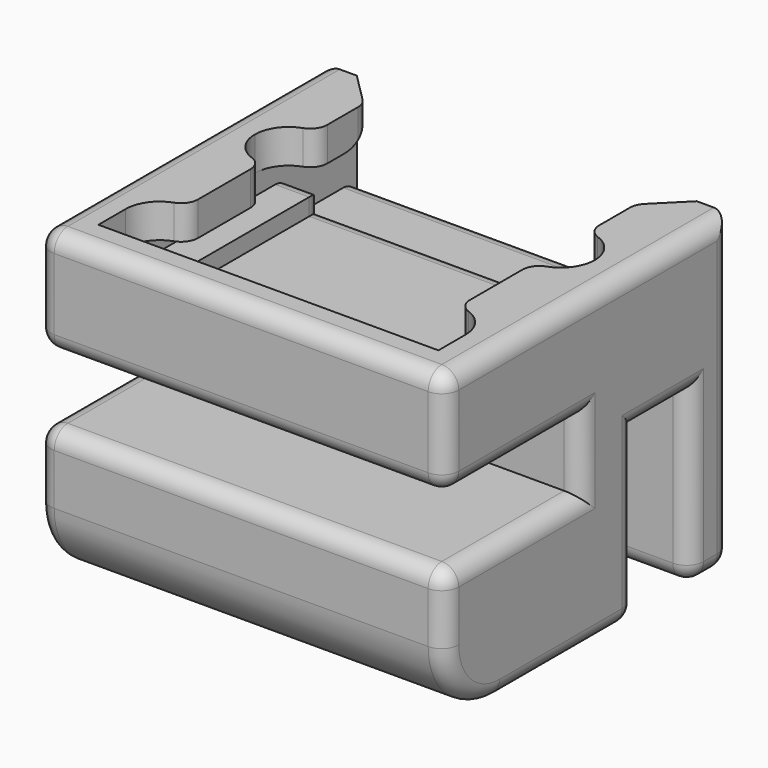
from build123d import *

# Parameters (mm, degrees)
F0_W           = 30.48
F0_H           = 26.67
F1_DEPTH       = 19.05
F3_DEPTH       = 1.524
F5_DEPTH       = 2.54
F6_W           = 20.32
F6_H           = 24.13
F7_DEPTH       = 1.27
F8_W           = 25.4
F8_H           = 6.35
F9_DEPTH       = 2.794
F10_W          = 12.7
F10_H          = 5.08
F10_W_2        = 5.08
F10_H_2        = 12.7
F11_DEPTH      = 30.481
F12_R          = 5.08
F13_T1_DEPTH   = 27.94
F13_T3_DEPTH   = 3.81
F13_T5_DEPTH   = 11.43
F13_T7_DEPTH   = 11.43
F13_T9_DEPTH   = 5.08
F13_T11_DEPTH  = 11.43
F13_T13_DEPTH  = 5.08
F13_T15_DEPTH  = 5.334
F13_T17_DEPTH  = 25.4
F13_T19_DEPTH  = 1.27
F13_T21_DEPTH  = 21.844
F13_T23_DEPTH  = 25.4
F13_T25_DEPTH  = 20.32
F13_T27_DEPTH  = 2.54
F13_T29_DEPTH  = 1.27
F13_T31_DEPTH  = 2.54
F13_T33_DEPTH  = 2.54
F13_S37_W      = 1.2954
F13_S37_H      = 1.2954
F13_T38_DEPTH  = 1.2954
F13_S43_W      = 1.2954
F13_S43_H      = 1.2954
F13_T44_DEPTH  = 1.2954
F13_S49_W      = 1.2954
F13_S49_H      = 1.2954
F13_T50_DEPTH  = 1.2954
F13_S55_W      = 1.2954
F13_S55_H      = 1.2954
F13_T56_DEPTH  = 1.2954
F13_S61_W      = 1.2954
F13_S61_H      = 1.2954
F13_T62_DEPTH  = 1.2954
F13_S67_W      = 1.2954
F13_S67_H      = 1.2954
F13_T68_DEPTH  = 1.2954
F13_S73_W      = 1.2954
F13_S73_H      = 1.2954
F13_T74_DEPTH  = 1.2954
F13_S79_W      = 1.2954
F13_S79_H      = 1.2954
F13_T80_DEPTH  = 1.2954
F13_S85_W      = 1.2954
F13_S85_H      = 1.2954
F13_T86_DEPTH  = 1.2954
F13_S91_W      = 1.2954
F13_S91_H      = 1.2954
F13_T92_DEPTH  = 1.2954
F13_S97_W      = 1.2954
F13_S97_H      = 1.2954
F13_T98_DEPTH  = 1.2954
F13_S103_W     = 1.2954
F13_S103_H     = 1.2954
F13_T104_DEPTH = 1.2954
F13_T108_ANGLE = 90
F13_T110_ANGLE = 90
F13_T114_DEPTH = 9.9421024484
F13_T121_DEPTH = 9.9421024484
F13_T129_DEPTH = 14.605
F13_T133_DEPTH = 8.255
F13_T140_DEPTH = 8.255
F13_T144_DEPTH = 14.605
F13_T151_DEPTH = 14.605
F13_T155_DEPTH = 8.255
F13_T162_DEPTH = 8.255
F13_T166_DEPTH = 14.605
F13_T173_DEPTH = 28.575
F13_T177_DEPTH = 25.019
F13_T184_DEPTH = 14.605
F13_T188_DEPTH = 8.255
F13_T195_DEPTH = 8.255
F13_T199_DEPTH = 14.605
F13_T206_DEPTH = 14.605
F13_T210_DEPTH = 8.255
F13_T217_DEPTH = 8.255
F13_T221_DEPTH = 14.605
F13_T228_DEPTH = 28.575
F13_T232_DEPTH = 25.019
F13_T239_DEPTH = 4.445
F13_T243_DEPTH = 23.495
F13_T250_DEPTH = 23.495
F13_T254_DEPTH = 4.445
F13_T261_DEPTH = 5.715
F13_T265_DEPTH = 4.445
F13_T272_DEPTH = 5.715
F13_T276_DEPTH = 4.445
F13_T283_DEPTH = 3.8551280605
F13_T287_DEPTH = 9.9421024484
F13_T294_DEPTH = 3.8551280605
F13_T298_DEPTH = 9.9421024484


# Not quite as in the source:
# - a fillet or chamfer that OpenCascade refuses, or shapes differently, is made with other operations: its cross-section is extruded or revolved along the edge and cut away or added


with BuildPart() as f1:
    # F0 (on Top) → F1 (new body)
    with BuildSketch(Plane.XY):
        Rectangle(F0_W, F0_H)
    extrude(amount=F1_DEPTH)

    # F2 (on face) → F3 (join)
    with BuildSketch(Plane.XY.offset(19.05)):
        Polygon((-12.7, 13.335), (-15.24, 13.335), (-15.24, -13.335), (15.24, -13.335), (15.24, 13.335), (12.7, 13.335), (12.7, -10.795), (-12.7, -10.795), align=None)
    extrude(amount=F3_DEPTH)

    # F4 (on face) → F5 (join)
    with BuildSketch(Plane.XY.offset(20.574)):
        with BuildLine():
            ThreePointArc((-10.16, 1.27), (-11.9560512242, 2.0139487758), (-12.7, 3.81))
            Line((-12.7, 3.81), (-12.7, -8.255))
            ThreePointArc((-12.7, -8.255), (-11.9560512242, -6.4589487758), (-10.16, -5.715))
            Line((-10.16, -5.715), (-10.16, 1.27))
        make_face()
        with BuildLine():
            Line((-10.16, 10.795), (-12.7, 13.335))
            Line((-12.7, 13.335), (-12.7, 3.81))
            ThreePointArc((-12.7, 3.81), (-11.9560512242, 5.6060512242), (-10.16, 6.35))
            Line((-10.16, 6.35), (-10.16, 10.795))
        make_face()
        Polygon((15.24, -13.335), (15.24, 13.335), (12.7, 13.335), (12.7, 3.81), (12.7, -8.255), (12.7, -10.795), (0, -10.795), (-12.7, -10.795), (-12.7, -8.255), (-12.7, 3.81), (-12.7, 13.335), (-15.24, 13.335), (-15.24, -13.335), align=None)
        with BuildLine():
            Line((12.7, -8.255), (12.7, 3.81))
            ThreePointArc((12.7, 3.81), (11.9560512242, 2.0139487758), (10.16, 1.27))
            Line((10.16, 1.27), (10.16, -5.715))
            ThreePointArc((10.16, -5.715), (11.9560512242, -6.4589487758), (12.7, -8.255))
        make_face()
        with BuildLine():
            Line((12.7, 3.81), (12.7, 13.335))
            Line((12.7, 13.335), (10.16, 10.795))
            Line((10.16, 10.795), (10.16, 6.35))
            ThreePointArc((10.16, 6.35), (11.9560512242, 5.6060512242), (12.7, 3.81))
        make_face()
    extrude(amount=F5_DEPTH)

    # F6 (on face) → F7 (cut)
    with BuildSketch(Plane.XY.offset(19.05)):
        with Locations((0, 1.27)):
            Rectangle(F6_W, F6_H)
    extrude(amount=-F7_DEPTH, mode=Mode.SUBTRACT)

    # F8 (on face) → F9 (cut)
    with BuildSketch(Plane.XY.offset(19.05)):
        with Locations((0, 10.16)):
            Rectangle(F8_W, F8_H)
    extrude(amount=-F9_DEPTH, mode=Mode.SUBTRACT)

    # F10 (on face) → F11 (cut, through all)
    with BuildSketch(Plane.YZ.offset(15.24)):
        with Locations((-6.985, 12.7)):
            Rectangle(F10_W, F10_H)
        with Locations((6.985, 6.35)):
            Rectangle(F10_W_2, F10_H_2)
    extrude(amount=-F11_DEPTH, mode=Mode.SUBTRACT)

    # F12
    f12_edges = [f1.edges().sort_by_distance(p)[0] for p in [
        (0, -13.335, 0),
    ]]
    fillet(f12_edges, radius=F12_R)

    # F13: fillet of radius 1.27 on 48 edges, made by hand

    # F13_s2 → F13_t1 (cut)
    with BuildSketch(Plane.YZ.offset(-13.97)):
        with BuildLine():
            ThreePointArc((-13.335, 8.89), (-12.9630256121, 9.7880256121), (-12.065, 10.16))
            Line((-12.065, 10.16), (-12.065, 10.1854))
            Line((-12.065, 10.1854), (-13.3604, 10.1854))
            Line((-13.3604, 10.1854), (-13.3604, 8.89))
            Line((-13.3604, 8.89), (-13.335, 8.89))
        make_face()
        with BuildLine():
            ThreePointArc((-12.065, 15.24), (-12.9630256121, 15.6119743879), (-13.335, 16.51))
            Line((-13.335, 16.51), (-13.3604, 16.51))
            Line((-13.3604, 16.51), (-13.3604, 15.2146))
            Line((-13.3604, 15.2146), (-12.065, 15.2146))
            Line((-12.065, 15.2146), (-12.065, 15.24))
        make_face()
        with BuildLine():
            ThreePointArc((3.175, 0), (4.0730256121, 0.3719743879), (4.445, 1.27))
            Line((4.445, 1.27), (4.4704, 1.27))
            Line((4.4704, 1.27), (4.4704, -0.0254))
            Line((4.4704, -0.0254), (3.175, -0.0254))
            Line((3.175, -0.0254), (3.175, 0))
        make_face()
        with BuildLine():
            ThreePointArc((9.525, 1.27), (9.8969743879, 0.3719743879), (10.795, 0))
            Line((10.795, 0), (10.795, -0.0254))
            Line((10.795, -0.0254), (9.4996, -0.0254))
            Line((9.4996, -0.0254), (9.4996, 1.27))
            Line((9.4996, 1.27), (9.525, 1.27))
        make_face()
        with BuildLine():
            ThreePointArc((12.065, 0), (12.9630256121, 0.3719743879), (13.335, 1.27))
            Line((13.335, 1.27), (13.3604, 1.27))
            Line((13.3604, 1.27), (13.3604, -0.0254))
            Line((13.3604, -0.0254), (12.065, -0.0254))
            Line((12.065, -0.0254), (12.065, 0))
        make_face()
        with BuildLine():
            ThreePointArc((-13.335, 21.844), (-12.9630256121, 22.7420256121), (-12.065, 23.114))
            Line((-12.065, 23.114), (-12.065, 23.1394))
            Line((-12.065, 23.1394), (-13.3604, 23.1394))
            Line((-13.3604, 23.1394), (-13.3604, 21.844))
            Line((-13.3604, 21.844), (-13.335, 21.844))
        make_face()
    extrude(amount=F13_T1_DEPTH, mode=Mode.SUBTRACT)

    # F13_s4 → F13_t3 (cut)
    with BuildSketch(Plane.XY.offset(5.08)):
        with BuildLine():
            ThreePointArc((15.24, -12.065), (14.8680256121, -12.9630256121), (13.97, -13.335))
            Line((13.97, -13.335), (13.97, -13.3604))
            Line((13.97, -13.3604), (15.2654, -13.3604))
            Line((15.2654, -13.3604), (15.2654, -12.065))
            Line((15.2654, -12.065), (15.24, -12.065))
        make_face()
        with BuildLine():
            ThreePointArc((-13.97, -13.335), (-14.8680256121, -12.9630256121), (-15.24, -12.065))
            Line((-15.24, -12.065), (-15.2654, -12.065))
            Line((-15.2654, -12.065), (-15.2654, -13.3604))
            Line((-15.2654, -13.3604), (-13.97, -13.3604))
            Line((-13.97, -13.3604), (-13.97, -13.335))
        make_face()
    extrude(amount=F13_T3_DEPTH, mode=Mode.SUBTRACT)

    # F13_s6 → F13_t5 (cut)
    with BuildSketch(Plane.XZ.offset(0.635)):
        with BuildLine():
            ThreePointArc((15.24, 8.89), (14.8680256121, 9.7880256121), (13.97, 10.16))
            Line((13.97, 10.16), (13.97, 10.1854))
            Line((13.97, 10.1854), (15.2654, 10.1854))
            Line((15.2654, 10.1854), (15.2654, 8.89))
            Line((15.2654, 8.89), (15.24, 8.89))
        make_face()
        with BuildLine():
            ThreePointArc((15.24, 16.51), (14.8680256121, 15.6119743879), (13.97, 15.24))
            Line((13.97, 15.24), (13.97, 15.2146))
            Line((13.97, 15.2146), (15.2654, 15.2146))
            Line((15.2654, 15.2146), (15.2654, 16.51))
            Line((15.2654, 16.51), (15.24, 16.51))
        make_face()
        with BuildLine():
            ThreePointArc((-13.97, 10.16), (-14.8680256121, 9.7880256121), (-15.24, 8.89))
            Line((-15.24, 8.89), (-15.2654, 8.89))
            Line((-15.2654, 8.89), (-15.2654, 10.1854))
            Line((-15.2654, 10.1854), (-13.97, 10.1854))
            Line((-13.97, 10.1854), (-13.97, 10.16))
        make_face()
        with BuildLine():
            ThreePointArc((-13.97, 15.24), (-14.8680256121, 15.6119743879), (-15.24, 16.51))
            Line((-15.24, 16.51), (-15.2654, 16.51))
            Line((-15.2654, 16.51), (-15.2654, 15.2146))
            Line((-15.2654, 15.2146), (-13.97, 15.2146))
            Line((-13.97, 15.2146), (-13.97, 15.24))
        make_face()
    extrude(amount=F13_T5_DEPTH, mode=Mode.SUBTRACT)

    # F13_s8 → F13_t7 (cut)
    with BuildSketch(Plane.XZ.offset(-3.175)):
        with BuildLine():
            ThreePointArc((15.24, 1.27), (14.8680256121, 0.3719743879), (13.97, 0))
            Line((13.97, 0), (13.97, -0.0254))
            Line((13.97, -0.0254), (15.2654, -0.0254))
            Line((15.2654, -0.0254), (15.2654, 1.27))
            Line((15.2654, 1.27), (15.24, 1.27))
        make_face()
        with BuildLine():
            ThreePointArc((-13.97, 0), (-14.8680256121, 0.3719743879), (-15.24, 1.27))
            Line((-15.24, 1.27), (-15.2654, 1.27))
            Line((-15.2654, 1.27), (-15.2654, -0.0254))
            Line((-15.2654, -0.0254), (-13.97, -0.0254))
            Line((-13.97, -0.0254), (-13.97, 0))
        make_face()
    extrude(amount=F13_T7_DEPTH, mode=Mode.SUBTRACT)

    # F13_s10 → F13_t9 (cut)
    with BuildSketch(Plane.XY.offset(10.16)):
        with BuildLine():
            ThreePointArc((15.24, 0.635), (14.8680256121, -0.2630256121), (13.97, -0.635))
            Line((13.97, -0.635), (13.97, -0.6604))
            Line((13.97, -0.6604), (15.2654, -0.6604))
            Line((15.2654, -0.6604), (15.2654, 0.635))
            Line((15.2654, 0.635), (15.24, 0.635))
        make_face()
        with BuildLine():
            ThreePointArc((-13.97, -0.635), (-14.8680256121, -0.2630256121), (-15.24, 0.635))
            Line((-15.24, 0.635), (-15.2654, 0.635))
            Line((-15.2654, 0.635), (-15.2654, -0.6604))
            Line((-15.2654, -0.6604), (-13.97, -0.6604))
            Line((-13.97, -0.6604), (-13.97, -0.635))
        make_face()
    extrude(amount=F13_T9_DEPTH, mode=Mode.SUBTRACT)

    # F13_s12 → F13_t11 (cut)
    with BuildSketch(Plane.XY.offset(1.27)):
        with BuildLine():
            ThreePointArc((15.24, 3.175), (14.8680256121, 4.0730256121), (13.97, 4.445))
            Line((13.97, 4.445), (13.97, 4.4704))
            Line((13.97, 4.4704), (15.2654, 4.4704))
            Line((15.2654, 4.4704), (15.2654, 3.175))
            Line((15.2654, 3.175), (15.24, 3.175))
        make_face()
        with BuildLine():
            ThreePointArc((15.24, 10.795), (14.8680256121, 9.8969743879), (13.97, 9.525))
            Line((13.97, 9.525), (13.97, 9.4996))
            Line((13.97, 9.4996), (15.2654, 9.4996))
            Line((15.2654, 9.4996), (15.2654, 10.795))
            Line((15.2654, 10.795), (15.24, 10.795))
        make_face()
        with BuildLine():
            ThreePointArc((-13.97, 4.445), (-14.8680256121, 4.0730256121), (-15.24, 3.175))
            Line((-15.24, 3.175), (-15.2654, 3.175))
            Line((-15.2654, 3.175), (-15.2654, 4.4704))
            Line((-15.2654, 4.4704), (-13.97, 4.4704))
            Line((-13.97, 4.4704), (-13.97, 4.445))
        make_face()
        with BuildLine():
            ThreePointArc((-13.97, 9.525), (-14.8680256121, 9.8969743879), (-15.24, 10.795))
            Line((-15.24, 10.795), (-15.2654, 10.795))
            Line((-15.2654, 10.795), (-15.2654, 9.4996))
            Line((-15.2654, 9.4996), (-13.97, 9.4996))
            Line((-13.97, 9.4996), (-13.97, 9.525))
        make_face()
    extrude(amount=F13_T11_DEPTH, mode=Mode.SUBTRACT)

    # F13_s14 → F13_t13 (cut)
    with BuildSketch(Plane.XZ.offset(-9.525)):
        with BuildLine():
            ThreePointArc((15.24, 13.97), (14.8680256121, 13.0719743879), (13.97, 12.7))
            Line((13.97, 12.7), (13.97, 12.6746))
            Line((13.97, 12.6746), (15.2654, 12.6746))
            Line((15.2654, 12.6746), (15.2654, 13.97))
            Line((15.2654, 13.97), (15.24, 13.97))
        make_face()
        with BuildLine():
            ThreePointArc((-13.97, 12.7), (-14.8680256121, 13.0719743879), (-15.24, 13.97))
            Line((-15.24, 13.97), (-15.2654, 13.97))
            Line((-15.2654, 13.97), (-15.2654, 12.6746))
            Line((-15.2654, 12.6746), (-13.97, 12.6746))
            Line((-13.97, 12.6746), (-13.97, 12.7))
        make_face()
    extrude(amount=F13_T13_DEPTH, mode=Mode.SUBTRACT)

    # F13_s16 → F13_t15 (cut)
    with BuildSketch(Plane.XY.offset(16.51)):
        with BuildLine():
            ThreePointArc((15.24, -12.065), (14.8680256121, -12.9630256121), (13.97, -13.335))
            Line((13.97, -13.335), (13.97, -13.3604))
            Line((13.97, -13.3604), (15.2654, -13.3604))
            Line((15.2654, -13.3604), (15.2654, -12.065))
            Line((15.2654, -12.065), (15.24, -12.065))
        make_face()
        with BuildLine():
            ThreePointArc((-13.97, -13.335), (-14.8680256121, -12.9630256121), (-15.24, -12.065))
            Line((-15.24, -12.065), (-15.2654, -12.065))
            Line((-15.2654, -12.065), (-15.2654, -13.3604))
            Line((-15.2654, -13.3604), (-13.97, -13.3604))
            Line((-13.97, -13.3604), (-13.97, -13.335))
        make_face()
    extrude(amount=F13_T15_DEPTH, mode=Mode.SUBTRACT)

    # F13_s18 → F13_t17 (cut)
    with BuildSketch(Plane.XZ.offset(-13.335)):
        with BuildLine():
            ThreePointArc((15.24, 21.844), (14.8680256121, 22.7420256121), (13.97, 23.114))
            Line((13.97, 23.114), (13.97, 23.1394))
            Line((13.97, 23.1394), (15.2654, 23.1394))
            Line((15.2654, 23.1394), (15.2654, 21.844))
            Line((15.2654, 21.844), (15.24, 21.844))
        make_face()
        with BuildLine():
            ThreePointArc((-13.97, 23.114), (-14.8680256121, 22.7420256121), (-15.24, 21.844))
            Line((-15.24, 21.844), (-15.2654, 21.844))
            Line((-15.2654, 21.844), (-15.2654, 23.1394))
            Line((-15.2654, 23.1394), (-13.97, 23.1394))
            Line((-13.97, 23.1394), (-13.97, 23.114))
        make_face()
    extrude(amount=F13_T17_DEPTH, mode=Mode.SUBTRACT)

    # F13_s20 → F13_t19 (cut)
    with BuildSketch(Plane.XZ.offset(-12.065)):
        with BuildLine():
            ThreePointArc((15.24, 1.27), (14.8680256121, 0.3719743879), (13.97, 0))
            Line((13.97, 0), (13.97, -0.0254))
            Line((13.97, -0.0254), (15.2654, -0.0254))
            Line((15.2654, -0.0254), (15.2654, 1.27))
            Line((15.2654, 1.27), (15.24, 1.27))
        make_face()
        with BuildLine():
            ThreePointArc((-13.97, 0), (-14.8680256121, 0.3719743879), (-15.24, 1.27))
            Line((-15.24, 1.27), (-15.2654, 1.27))
            Line((-15.2654, 1.27), (-15.2654, -0.0254))
            Line((-15.2654, -0.0254), (-13.97, -0.0254))
            Line((-13.97, -0.0254), (-13.97, 0))
        make_face()
    extrude(amount=F13_T19_DEPTH, mode=Mode.SUBTRACT)

    # F13_s22 → F13_t21 (cut)
    with BuildSketch(Plane.XY.offset(1.27)):
        with BuildLine():
            ThreePointArc((15.24, 12.065), (14.8680256121, 12.9630256121), (13.97, 13.335))
            Line((13.97, 13.335), (13.97, 13.3604))
            Line((13.97, 13.3604), (15.2654, 13.3604))
            Line((15.2654, 13.3604), (15.2654, 12.065))
            Line((15.2654, 12.065), (15.24, 12.065))
        make_face()
        with BuildLine():
            ThreePointArc((-13.97, 13.335), (-14.8680256121, 12.9630256121), (-15.24, 12.065))
            Line((-15.24, 12.065), (-15.2654, 12.065))
            Line((-15.2654, 12.065), (-15.2654, 13.3604))
            Line((-15.2654, 13.3604), (-13.97, 13.3604))
            Line((-13.97, 13.3604), (-13.97, 13.335))
        make_face()
    extrude(amount=F13_T21_DEPTH, mode=Mode.SUBTRACT)

    # F13_s24 → F13_t23 (cut)
    with BuildSketch(Plane.YZ.offset(-12.7)):
        with BuildLine():
            ThreePointArc((13.335, 14.986), (12.9630256121, 15.8840256121), (12.065, 16.256))
            Line((12.065, 16.256), (12.065, 16.2814))
            Line((12.065, 16.2814), (13.3604, 16.2814))
            Line((13.3604, 16.2814), (13.3604, 14.986))
            Line((13.3604, 14.986), (13.335, 14.986))
        make_face()
    extrude(amount=F13_T23_DEPTH, mode=Mode.SUBTRACT)

    # F13_s26 → F13_t25 (cut)
    with BuildSketch(Plane.YZ.offset(-10.16)):
        with BuildLine():
            ThreePointArc((6.985, 16.51), (6.6130256121, 17.4080256121), (5.715, 17.78))
            Line((5.715, 17.78), (5.715, 17.8054))
            Line((5.715, 17.8054), (7.0104, 17.8054))
            Line((7.0104, 17.8054), (7.0104, 16.51))
            Line((7.0104, 16.51), (6.985, 16.51))
        make_face()
    extrude(amount=F13_T25_DEPTH, mode=Mode.SUBTRACT)

    # F13_s28 → F13_t27 (cut)
    with BuildSketch(Plane.YZ.offset(10.16)):
        with BuildLine():
            ThreePointArc((5.715, 19.05), (6.6130256121, 18.6780256121), (6.985, 17.78))
            Line((6.985, 17.78), (7.0104, 17.78))
            Line((7.0104, 17.78), (7.0104, 19.0754))
            Line((7.0104, 19.0754), (5.715, 19.0754))
            Line((5.715, 19.0754), (5.715, 19.05))
        make_face()
    extrude(amount=F13_T27_DEPTH, mode=Mode.SUBTRACT)

    # F13_s30 → F13_t29 (cut)
    with BuildSketch(Plane.XY.offset(17.78)):
        with BuildLine():
            ThreePointArc((11.43, 6.985), (10.5319743879, 6.6130256121), (10.16, 5.715))
            Line((10.16, 5.715), (10.1346, 5.715))
            Line((10.1346, 5.715), (10.1346, 7.0104))
            Line((10.1346, 7.0104), (11.43, 7.0104))
            Line((11.43, 7.0104), (11.43, 6.985))
        make_face()
        with BuildLine():
            ThreePointArc((-11.43, 6.985), (-10.5319743879, 6.6130256121), (-10.16, 5.715))
            Line((-10.16, 5.715), (-10.1346, 5.715))
            Line((-10.1346, 5.715), (-10.1346, 7.0104))
            Line((-10.1346, 7.0104), (-11.43, 7.0104))
            Line((-11.43, 7.0104), (-11.43, 6.985))
        make_face()
    extrude(amount=F13_T29_DEPTH, mode=Mode.SUBTRACT)

    # F13_s32 → F13_t31 (cut)
    with BuildSketch(Plane.YZ.offset(-12.7)):
        with BuildLine():
            ThreePointArc((6.985, 17.78), (6.6130256121, 18.6780256121), (5.715, 19.05))
            Line((5.715, 19.05), (5.715, 19.0754))
            Line((5.715, 19.0754), (7.0104, 19.0754))
            Line((7.0104, 19.0754), (7.0104, 17.78))
            Line((7.0104, 17.78), (6.985, 17.78))
        make_face()
    extrude(amount=F13_T31_DEPTH, mode=Mode.SUBTRACT)

    # F13_s34 → F13_t33 (cut)
    with BuildSketch(Plane.XY.offset(20.574)):
        with BuildLine():
            ThreePointArc((-10.16, 10.2689487758), (-10.2566729937, 10.7549567349), (-10.5319743879, 11.1669743879))
            Line((-10.5319743879, 11.1669743879), (-10.5140138757, 11.1849349001))
            Line((-10.5140138757, 11.1849349001), (-10.1346, 10.8055210245))
            Line((-10.1346, 10.8055210245), (-10.1346, 10.2689487758))
            Line((-10.1346, 10.2689487758), (-10.16, 10.2689487758))
        make_face()
        with BuildLine():
            ThreePointArc((10.5319743879, 11.1669743879), (10.2566729937, 10.7549567349), (10.16, 10.2689487758))
            Line((10.16, 10.2689487758), (10.1346, 10.2689487758))
            Line((10.1346, 10.2689487758), (10.1346, 10.8055210245))
            Line((10.1346, 10.8055210245), (10.5140138757, 11.1849349001))
            Line((10.5140138757, 11.1849349001), (10.5319743879, 11.1669743879))
        make_face()
        with BuildLine():
            ThreePointArc((-11.0066666667, 6.2047349656), (-10.3930493422, 6.6688676066), (-10.16, 7.4021024484))
            Line((-10.16, 7.4021024484), (-10.1346, 7.4021024484))
            Line((-10.1346, 7.4021024484), (-10.1346, 6.35))
            Line((-10.1346, 6.35), (-10.16, 6.3246))
            ThreePointArc((-10.16, 6.3246), (-10.5852238357, 6.2883861381), (-10.9982, 6.180787616))
            Line((-10.9982, 6.180787616), (-11.0066666667, 6.2047349656))
        make_face()
        with BuildLine():
            ThreePointArc((10.16, 7.4021024484), (10.3930493422, 6.6688676066), (11.0066666667, 6.2047349656))
            Line((11.0066666667, 6.2047349656), (10.9982, 6.180787616))
            ThreePointArc((10.9982, 6.180787616), (10.5852238357, 6.2883861381), (10.16, 6.3246))
            Line((10.16, 6.3246), (10.1346, 6.35))
            Line((10.1346, 6.35), (10.1346, 7.4021024484))
            Line((10.1346, 7.4021024484), (10.16, 7.4021024484))
        make_face()
        with BuildLine():
            ThreePointArc((10.16, -4.6628975516), (10.3930493422, -5.3961323934), (11.0066666667, -5.8602650344))
            Line((11.0066666667, -5.8602650344), (10.9982, -5.884212384))
            ThreePointArc((10.9982, -5.884212384), (10.5852238357, -5.7766138619), (10.16, -5.7404))
            Line((10.16, -5.7404), (10.1346, -5.715))
            Line((10.1346, -5.715), (10.1346, -4.6628975516))
            Line((10.1346, -4.6628975516), (10.16, -4.6628975516))
        make_face()
        with BuildLine():
            ThreePointArc((-10.16, -4.6628975516), (-10.3930493422, -5.3961323934), (-11.0066666667, -5.8602650344))
            Line((-11.0066666667, -5.8602650344), (-10.9982, -5.884212384))
            ThreePointArc((-10.9982, -5.884212384), (-10.5852238357, -5.7766138619), (-10.16, -5.7404))
            Line((-10.16, -5.7404), (-10.1346, -5.715))
            Line((-10.1346, -5.715), (-10.1346, -4.6628975516))
            Line((-10.1346, -4.6628975516), (-10.16, -4.6628975516))
        make_face()
        with BuildLine():
            ThreePointArc((-10.16, 0.2178975516), (-10.3930493422, 0.9511323934), (-11.0066666667, 1.4152650344))
            Line((-11.0066666667, 1.4152650344), (-10.9982, 1.439212384))
            ThreePointArc((-10.9982, 1.439212384), (-10.5852238357, 1.3316138619), (-10.16, 1.2954))
            Line((-10.16, 1.2954), (-10.1346, 1.27))
            Line((-10.1346, 1.27), (-10.1346, 0.2178975516))
            Line((-10.1346, 0.2178975516), (-10.16, 0.2178975516))
        make_face()
        with BuildLine():
            ThreePointArc((11.0066666667, 1.4152650344), (10.3930493422, 0.9511323934), (10.16, 0.2178975516))
            Line((10.16, 0.2178975516), (10.1346, 0.2178975516))
            Line((10.1346, 0.2178975516), (10.1346, 1.27))
            Line((10.1346, 1.27), (10.16, 1.2954))
            ThreePointArc((10.16, 1.2954), (10.5852238357, 1.3316138619), (10.9982, 1.439212384))
            Line((10.9982, 1.439212384), (11.0066666667, 1.4152650344))
        make_face()
    extrude(amount=F13_T33_DEPTH, mode=Mode.SUBTRACT)


with BuildPart() as f13_tool36:
    # F13_s37 → F13_t38 (new body)
    with BuildSketch(Plane.YZ.offset(13.97)):
        with Locations((-12.7127, 9.5377)):
            Rectangle(F13_S37_W, F13_S37_H)
    extrude(amount=F13_T38_DEPTH)

    # F13_s39 → F13_t40 (revolve, cut)
    with BuildSketch(Plane(origin=(13.97, -12.065, 8.89), x_dir=(0, 0.7071067812, -0.7071067812), z_dir=(0, -0.7071067812, -0.7071067812))):
        with BuildLine():
            ThreePointArc((0, -1.27), (1.27, 0), (0, 1.27))
            Line((0, 1.27), (0, -1.27))
        make_face()
    revolve(axis=Axis((13.97, -12.065, 8.89), (1, 0, 0)), mode=Mode.SUBTRACT)


with BuildPart() as f1_1:
    add(f1.part)

    # F13_t35: cut F13_tool36
    add(f13_tool36.part, mode=Mode.SUBTRACT)


with BuildPart() as f13_tool42:
    # F13_s43 → F13_t44 (new body)
    with BuildSketch(Plane.XZ.offset(12.065)):
        with Locations((-14.6177, 9.5377)):
            Rectangle(F13_S43_W, F13_S43_H)
    extrude(amount=F13_T44_DEPTH)

    # F13_s45 → F13_t46 (revolve, cut)
    with BuildSketch(Plane(origin=(-13.97, -12.065, 8.89), x_dir=(0.7071067812, 0, -0.7071067812), z_dir=(-0.7071067812, 0, -0.7071067812))):
        with BuildLine():
            ThreePointArc((0, -1.27), (1.27, 0), (0, 1.27))
            Line((0, 1.27), (0, -1.27))
        make_face()
    revolve(axis=Axis((-13.97, -12.065, 8.89), (0, -1, 0)), mode=Mode.SUBTRACT)


with BuildPart() as f1_2:
    add(f1_1.part)

    # F13_t41: cut F13_tool42
    add(f13_tool42.part, mode=Mode.SUBTRACT)


with BuildPart() as f13_tool48:
    # F13_s49 → F13_t50 (new body)
    with BuildSketch(Plane.YZ.offset(13.97)):
        with Locations((-12.7127, 15.8623)):
            Rectangle(F13_S49_W, F13_S49_H)
    extrude(amount=F13_T50_DEPTH)

    # F13_s51 → F13_t52 (revolve, cut)
    with BuildSketch(Plane(origin=(13.97, -12.065, 16.51), x_dir=(0, 0.7071067812, 0.7071067812), z_dir=(0, 0.7071067812, -0.7071067812))):
        with BuildLine():
            ThreePointArc((0, -1.27), (1.27, 0), (0, 1.27))
            Line((0, 1.27), (0, -1.27))
        make_face()
    revolve(axis=Axis((13.97, -12.065, 16.51), (1, 0, 0)), mode=Mode.SUBTRACT)


with BuildPart() as f1_3:
    add(f1_2.part)

    # F13_t47: cut F13_tool48
    add(f13_tool48.part, mode=Mode.SUBTRACT)


with BuildPart() as f13_tool54:
    # F13_s55 → F13_t56 (new body)
    with BuildSketch(Plane.XZ.offset(12.065)):
        with Locations((-14.6177, 15.8623)):
            Rectangle(F13_S55_W, F13_S55_H)
    extrude(amount=F13_T56_DEPTH)

    # F13_s57 → F13_t58 (revolve, cut)
    with BuildSketch(Plane(origin=(-13.97, -12.065, 16.51), x_dir=(0.7071067812, 0, 0.7071067812), z_dir=(0.7071067812, 0, -0.7071067812))):
        with BuildLine():
            ThreePointArc((0, -1.27), (1.27, 0), (0, 1.27))
            Line((0, 1.27), (0, -1.27))
        make_face()
    revolve(axis=Axis((-13.97, -12.065, 16.51), (0, -1, 0)), mode=Mode.SUBTRACT)


with BuildPart() as f1_4:
    add(f1_3.part)

    # F13_t53: cut F13_tool54
    add(f13_tool54.part, mode=Mode.SUBTRACT)


with BuildPart() as f13_tool60:
    # F13_s61 → F13_t62 (new body)
    with BuildSketch(Plane.YZ.offset(13.97)):
        with Locations((3.8227, 0.6223)):
            Rectangle(F13_S61_W, F13_S61_H)
    extrude(amount=F13_T62_DEPTH)

    # F13_s63 → F13_t64 (revolve, cut)
    with BuildSketch(Plane(origin=(13.97, 3.175, 1.27), x_dir=(0, -0.7071067812, 0.7071067812), z_dir=(0, 0.7071067812, 0.7071067812))):
        with BuildLine():
            ThreePointArc((0, -1.27), (1.27, 0), (0, 1.27))
            Line((0, 1.27), (0, -1.27))
        make_face()
    revolve(axis=Axis((13.97, 3.175, 1.27), (1, 0, 0)), mode=Mode.SUBTRACT)


with BuildPart() as f1_5:
    add(f1_4.part)

    # F13_t59: cut F13_tool60
    add(f13_tool60.part, mode=Mode.SUBTRACT)


with BuildPart() as f13_tool66:
    # F13_s67 → F13_t68 (new body)
    with BuildSketch(Plane.XY.offset(1.27)):
        with Locations((-14.6177, 3.8227)):
            Rectangle(F13_S67_W, F13_S67_H)
    extrude(amount=-F13_T68_DEPTH)

    # F13_s69 → F13_t70 (revolve, cut)
    with BuildSketch(Plane(origin=(-13.97, 3.175, 1.27), x_dir=(0.7071067812, -0.7071067812, 0), z_dir=(0.7071067812, 0.7071067812, 0))):
        with BuildLine():
            ThreePointArc((0, -1.27), (1.27, 0), (0, 1.27))
            Line((0, 1.27), (0, -1.27))
        make_face()
    revolve(axis=Axis((-13.97, 3.175, 1.27), (0, 0, -1)), mode=Mode.SUBTRACT)


with BuildPart() as f1_6:
    add(f1_5.part)

    # F13_t65: cut F13_tool66
    add(f13_tool66.part, mode=Mode.SUBTRACT)


with BuildPart() as f13_tool72:
    # F13_s73 → F13_t74 (new body)
    with BuildSketch(Plane.YZ.offset(13.97)):
        with Locations((10.1473, 0.6223)):
            Rectangle(F13_S73_W, F13_S73_H)
    extrude(amount=F13_T74_DEPTH)

    # F13_s75 → F13_t76 (revolve, cut)
    with BuildSketch(Plane(origin=(13.97, 10.795, 1.27), x_dir=(0, 0.7071067812, 0.7071067812), z_dir=(0, 0.7071067812, -0.7071067812))):
        with BuildLine():
            ThreePointArc((0, -1.27), (1.27, 0), (0, 1.27))
            Line((0, 1.27), (0, -1.27))
        make_face()
    revolve(axis=Axis((13.97, 10.795, 1.27), (1, 0, 0)), mode=Mode.SUBTRACT)


with BuildPart() as f1_7:
    add(f1_6.part)

    # F13_t71: cut F13_tool72
    add(f13_tool72.part, mode=Mode.SUBTRACT)


with BuildPart() as f13_tool78:
    # F13_s79 → F13_t80 (new body)
    with BuildSketch(Plane.XZ.offset(-10.795)):
        with Locations((-14.6177, 0.6223)):
            Rectangle(F13_S79_W, F13_S79_H)
    extrude(amount=F13_T80_DEPTH)

    # F13_s81 → F13_t82 (revolve, cut)
    with BuildSketch(Plane(origin=(-13.97, 10.795, 1.27), x_dir=(0.7071067812, 0, 0.7071067812), z_dir=(0.7071067812, 0, -0.7071067812))):
        with BuildLine():
            ThreePointArc((0, -1.27), (1.27, 0), (0, 1.27))
            Line((0, 1.27), (0, -1.27))
        make_face()
    revolve(axis=Axis((-13.97, 10.795, 1.27), (0, -1, 0)), mode=Mode.SUBTRACT)


with BuildPart() as f1_8:
    add(f1_7.part)

    # F13_t77: cut F13_tool78
    add(f13_tool78.part, mode=Mode.SUBTRACT)


with BuildPart() as f13_tool84:
    # F13_s85 → F13_t86 (new body)
    with BuildSketch(Plane.YZ.offset(13.97)):
        with Locations((-12.7127, 22.4917)):
            Rectangle(F13_S85_W, F13_S85_H)
    extrude(amount=F13_T86_DEPTH)

    # F13_s87 → F13_t88 (revolve, cut)
    with BuildSketch(Plane(origin=(13.97, -12.065, 21.844), x_dir=(0, 0.7071067812, -0.7071067812), z_dir=(0, -0.7071067812, -0.7071067812))):
        with BuildLine():
            ThreePointArc((0, -1.27), (1.27, 0), (0, 1.27))
            Line((0, 1.27), (0, -1.27))
        make_face()
    revolve(axis=Axis((13.97, -12.065, 21.844), (1, 0, 0)), mode=Mode.SUBTRACT)


with BuildPart() as f1_9:
    add(f1_8.part)

    # F13_t83: cut F13_tool84
    add(f13_tool84.part, mode=Mode.SUBTRACT)


with BuildPart() as f13_tool90:
    # F13_s91 → F13_t92 (new body)
    with BuildSketch(Plane.YZ.offset(13.97)):
        with Locations((12.7127, 0.6223)):
            Rectangle(F13_S91_W, F13_S91_H)
    extrude(amount=F13_T92_DEPTH)

    # F13_s93 → F13_t94 (revolve, cut)
    with BuildSketch(Plane(origin=(13.97, 12.065, 1.27), x_dir=(0, -0.7071067812, 0.7071067812), z_dir=(0, 0.7071067812, 0.7071067812))):
        with BuildLine():
            ThreePointArc((0, -1.27), (1.27, 0), (0, 1.27))
            Line((0, 1.27), (0, -1.27))
        make_face()
    revolve(axis=Axis((13.97, 12.065, 1.27), (1, 0, 0)), mode=Mode.SUBTRACT)


with BuildPart() as f1_10:
    add(f1_9.part)

    # F13_t89: cut F13_tool90
    add(f13_tool90.part, mode=Mode.SUBTRACT)


with BuildPart() as f13_tool96:
    # F13_s97 → F13_t98 (new body)
    with BuildSketch(Plane.XY.offset(1.27)):
        with Locations((-14.6177, 12.7127)):
            Rectangle(F13_S97_W, F13_S97_H)
    extrude(amount=-F13_T98_DEPTH)

    # F13_s99 → F13_t100 (revolve, cut)
    with BuildSketch(Plane(origin=(-13.97, 12.065, 1.27), x_dir=(0.7071067812, -0.7071067812, 0), z_dir=(0.7071067812, 0.7071067812, 0))):
        with BuildLine():
            ThreePointArc((0, -1.27), (1.27, 0), (0, 1.27))
            Line((0, 1.27), (0, -1.27))
        make_face()
    revolve(axis=Axis((-13.97, 12.065, 1.27), (0, 0, -1)), mode=Mode.SUBTRACT)


with BuildPart() as f1_11:
    add(f1_10.part)

    # F13_t95: cut F13_tool96
    add(f13_tool96.part, mode=Mode.SUBTRACT)


with BuildPart() as f13_tool102:
    # F13_s103 → F13_t104 (new body)
    with BuildSketch(Plane.XZ.offset(12.065)):
        with Locations((-14.6177, 22.4917)):
            Rectangle(F13_S103_W, F13_S103_H)
    extrude(amount=F13_T104_DEPTH)

    # F13_s105 → F13_t106 (revolve, cut)
    with BuildSketch(Plane(origin=(-13.97, -12.065, 21.844), x_dir=(0.7071067812, 0, -0.7071067812), z_dir=(-0.7071067812, 0, -0.7071067812))):
        with BuildLine():
            ThreePointArc((0, -1.27), (1.27, 0), (0, 1.27))
            Line((0, 1.27), (0, -1.27))
        make_face()
    revolve(axis=Axis((-13.97, -12.065, 21.844), (0, -1, 0)), mode=Mode.SUBTRACT)


with BuildPart() as f1_12:
    add(f1_11.part)

    # F13_t101: cut F13_tool102
    add(f13_tool102.part, mode=Mode.SUBTRACT)

    # F13_s107 → F13_t108 (revolve, cut)
    with BuildSketch(Plane.XY.offset(5.08)):
        with BuildLine():
            ThreePointArc((15.24, -12.065), (14.8680256121, -12.9630256121), (13.97, -13.335))
            Line((13.97, -13.335), (13.97, -13.3604))
            Line((13.97, -13.3604), (15.2654, -13.3604))
            Line((15.2654, -13.3604), (15.2654, -12.065))
            Line((15.2654, -12.065), (15.24, -12.065))
        make_face()
    revolve(axis=Axis((15.24, -8.255, 5.08), (1, 0, 0)), revolution_arc=F13_T108_ANGLE, mode=Mode.SUBTRACT)

    # F13_s109 → F13_t110 (revolve, cut)
    with BuildSketch(Plane.XY.offset(5.08)):
        with BuildLine():
            ThreePointArc((-13.97, -13.335), (-14.8680256121, -12.9630256121), (-15.24, -12.065))
            Line((-15.24, -12.065), (-15.2654, -12.065))
            Line((-15.2654, -12.065), (-15.2654, -13.3604))
            Line((-15.2654, -13.3604), (-13.97, -13.3604))
            Line((-13.97, -13.3604), (-13.97, -13.335))
        make_face()
    revolve(axis=Axis((-15.24, -8.255, 5.08), (1, 0, 0)), revolution_arc=F13_T110_ANGLE, mode=Mode.SUBTRACT)


with BuildPart() as f13_tool112:
    # F13_s113 → F13_t114 (new body)
    with BuildSketch(Plane(origin=(-8.2324359697, 8.2324359697, 0), x_dir=(0, 0, 1), z_dir=(-0.7071067812, 0.7071067812, 0))):
        with BuildLine():
            ThreePointArc((21.844, 0.4490128061), (20.9459743879, 0.0770384182), (20.574, -0.8209871939))
            Line((20.574, -0.8209871939), (20.5486, -0.8209871939))
            Line((20.5486, -0.8209871939), (20.5486, 0.4744128061))
            Line((20.5486, 0.4744128061), (21.844, 0.4744128061))
            Line((21.844, 0.4744128061), (21.844, 0.4490128061))
        make_face()
    extrude(amount=F13_T114_DEPTH)

    split(bisect_by=Plane.XZ.offset(-13.335), keep=Keep.TOP)

    split(bisect_by=Plane.YZ.offset(-10.16), keep=Keep.BOTTOM)

    split(bisect_by=Plane.YZ.offset(-12.7), keep=Keep.TOP)


with BuildPart() as f1_13:
    add(f1_12.part)

    # F13_t111: cut F13_tool112
    add(f13_tool112.part, mode=Mode.SUBTRACT)


with BuildPart() as f13_tool119:
    # F13_s120 → F13_t121 (new body)
    with BuildSketch(Plane(origin=(15.2625640303, 15.2625640303, 0), x_dir=(0, 0, 1), z_dir=(-0.7071067812, -0.7071067812, 0))):
        with BuildLine():
            ThreePointArc((21.844, 0.4490128061), (20.9459743879, 0.0770384182), (20.574, -0.8209871939))
            Line((20.574, -0.8209871939), (20.5486, -0.8209871939))
            Line((20.5486, -0.8209871939), (20.5486, 0.4744128061))
            Line((20.5486, 0.4744128061), (21.844, 0.4744128061))
            Line((21.844, 0.4744128061), (21.844, 0.4490128061))
        make_face()
    extrude(amount=F13_T121_DEPTH)

    split(bisect_by=Plane.XZ.offset(-13.335), keep=Keep.TOP)

    split(bisect_by=Plane.YZ.offset(10.16), keep=Keep.TOP)

    split(bisect_by=Plane.YZ.offset(12.7), keep=Keep.BOTTOM)


with BuildPart() as f1_14:
    add(f1_13.part)

    # F13_t118: cut F13_tool119
    add(f13_tool119.part, mode=Mode.SUBTRACT)


with BuildPart() as f13_tool127:
    # F13_s128 → F13_t129 (new body)
    with BuildSketch(Plane.XZ.offset(12.065)):
        with BuildLine():
            ThreePointArc((15.24, 8.89), (14.8680256121, 9.7880256121), (13.97, 10.16))
            Line((13.97, 10.16), (13.97, 10.1854))
            Line((13.97, 10.1854), (15.2654, 10.1854))
            Line((15.2654, 10.1854), (15.2654, 8.89))
            Line((15.2654, 8.89), (15.24, 8.89))
        make_face()
    extrude(amount=-F13_T129_DEPTH)

    split(bisect_by=Plane.XZ.offset(0.635), keep=Keep.BOTTOM)


with BuildPart() as f13_tool131:
    # F13_s132 → F13_t133 (new body)
    with BuildSketch(Plane.XY.offset(6.985)):
        with BuildLine():
            ThreePointArc((15.24, 0.635), (14.8680256121, -0.2630256121), (13.97, -0.635))
            Line((13.97, -0.635), (13.97, -0.6604))
            Line((13.97, -0.6604), (15.2654, -0.6604))
            Line((15.2654, -0.6604), (15.2654, 0.635))
            Line((15.2654, 0.635), (15.24, 0.635))
        make_face()
    extrude(amount=F13_T133_DEPTH)

    split(bisect_by=Plane.XY.offset(10.16), keep=Keep.BOTTOM)


with BuildPart() as f13_tool127_1:
    add(f13_tool127.part)

    # F13_t135: intersect F13_tool131
    add(f13_tool131.part, mode=Mode.INTERSECT)


with BuildPart() as f1_15:
    add(f1_14.part)

    # F13_t125: cut F13_tool127
    add(f13_tool127_1.part, mode=Mode.SUBTRACT)


with BuildPart() as f13_tool138:
    # F13_s139 → F13_t140 (new body)
    with BuildSketch(Plane.XY.offset(10.16)):
        with BuildLine():
            ThreePointArc((15.24, 0.635), (14.8680256121, -0.2630256121), (13.97, -0.635))
            Line((13.97, -0.635), (13.97, -0.6604))
            Line((13.97, -0.6604), (15.2654, -0.6604))
            Line((15.2654, -0.6604), (15.2654, 0.635))
            Line((15.2654, 0.635), (15.24, 0.635))
        make_face()
    extrude(amount=F13_T140_DEPTH)

    split(bisect_by=Plane.XY.offset(15.24), keep=Keep.TOP)


with BuildPart() as f13_tool142:
    # F13_s143 → F13_t144 (new body)
    with BuildSketch(Plane.XZ.offset(-2.54)):
        with BuildLine():
            ThreePointArc((15.24, 16.51), (14.8680256121, 15.6119743879), (13.97, 15.24))
            Line((13.97, 15.24), (13.97, 15.2146))
            Line((13.97, 15.2146), (15.2654, 15.2146))
            Line((15.2654, 15.2146), (15.2654, 16.51))
            Line((15.2654, 16.51), (15.24, 16.51))
        make_face()
    extrude(amount=F13_T144_DEPTH)

    split(bisect_by=Plane.XZ.offset(0.635), keep=Keep.BOTTOM)


with BuildPart() as f13_tool138_1:
    add(f13_tool138.part)

    # F13_t146: intersect F13_tool142
    add(f13_tool142.part, mode=Mode.INTERSECT)


with BuildPart() as f1_16:
    add(f1_15.part)

    # F13_t136: cut F13_tool138
    add(f13_tool138_1.part, mode=Mode.SUBTRACT)


with BuildPart() as f13_tool149:
    # F13_s150 → F13_t151 (new body)
    with BuildSketch(Plane.XY.offset(15.875)):
        with BuildLine():
            ThreePointArc((15.24, 3.175), (14.8680256121, 4.0730256121), (13.97, 4.445))
            Line((13.97, 4.445), (13.97, 4.4704))
            Line((13.97, 4.4704), (15.2654, 4.4704))
            Line((15.2654, 4.4704), (15.2654, 3.175))
            Line((15.2654, 3.175), (15.24, 3.175))
        make_face()
    extrude(amount=-F13_T151_DEPTH)

    split(bisect_by=Plane.XY.offset(12.7), keep=Keep.TOP)


with BuildPart() as f13_tool153:
    # F13_s154 → F13_t155 (new body)
    with BuildSketch(Plane.XZ.offset(-9.525)):
        with BuildLine():
            ThreePointArc((15.24, 13.97), (14.8680256121, 13.0719743879), (13.97, 12.7))
            Line((13.97, 12.7), (13.97, 12.6746))
            Line((13.97, 12.6746), (15.2654, 12.6746))
            Line((15.2654, 12.6746), (15.2654, 13.97))
            Line((15.2654, 13.97), (15.24, 13.97))
        make_face()
    extrude(amount=F13_T155_DEPTH)

    split(bisect_by=Plane.XZ.offset(-4.445), keep=Keep.TOP)


with BuildPart() as f13_tool149_1:
    add(f13_tool149.part)

    # F13_t157: intersect F13_tool153
    add(f13_tool153.part, mode=Mode.INTERSECT)


with BuildPart() as f1_17:
    add(f1_16.part)

    # F13_t147: cut F13_tool149
    add(f13_tool149_1.part, mode=Mode.SUBTRACT)


with BuildPart() as f13_tool160:
    # F13_s161 → F13_t162 (new body)
    with BuildSketch(Plane.XZ.offset(-12.7)):
        with BuildLine():
            ThreePointArc((15.24, 13.97), (14.8680256121, 13.0719743879), (13.97, 12.7))
            Line((13.97, 12.7), (13.97, 12.6746))
            Line((13.97, 12.6746), (15.2654, 12.6746))
            Line((15.2654, 12.6746), (15.2654, 13.97))
            Line((15.2654, 13.97), (15.24, 13.97))
        make_face()
    extrude(amount=F13_T162_DEPTH)

    split(bisect_by=Plane.XZ.offset(-9.525), keep=Keep.BOTTOM)


with BuildPart() as f13_tool164:
    # F13_s165 → F13_t166 (new body)
    with BuildSketch(Plane.XY.offset(1.27)):
        with BuildLine():
            ThreePointArc((15.24, 10.795), (14.8680256121, 9.8969743879), (13.97, 9.525))
            Line((13.97, 9.525), (13.97, 9.4996))
            Line((13.97, 9.4996), (15.2654, 9.4996))
            Line((15.2654, 9.4996), (15.2654, 10.795))
            Line((15.2654, 10.795), (15.24, 10.795))
        make_face()
    extrude(amount=F13_T166_DEPTH)

    split(bisect_by=Plane.XY.offset(12.7), keep=Keep.TOP)


with BuildPart() as f13_tool160_1:
    add(f13_tool160.part)

    # F13_t168: intersect F13_tool164
    add(f13_tool164.part, mode=Mode.INTERSECT)


with BuildPart() as f1_18:
    add(f1_17.part)

    # F13_t158: cut F13_tool160
    add(f13_tool160_1.part, mode=Mode.SUBTRACT)


with BuildPart() as f13_tool171:
    # F13_s172 → F13_t173 (new body)
    with BuildSketch(Plane.XZ.offset(12.065)):
        with BuildLine():
            ThreePointArc((15.24, 21.844), (14.8680256121, 22.7420256121), (13.97, 23.114))
            Line((13.97, 23.114), (13.97, 23.1394))
            Line((13.97, 23.1394), (15.2654, 23.1394))
            Line((15.2654, 23.1394), (15.2654, 21.844))
            Line((15.2654, 21.844), (15.24, 21.844))
        make_face()
    extrude(amount=-F13_T173_DEPTH)

    split(bisect_by=Plane.XZ.offset(-13.335), keep=Keep.BOTTOM)


with BuildPart() as f13_tool175:
    # F13_s176 → F13_t177 (new body)
    with BuildSketch(Plane.XY.offset(1.27)):
        with BuildLine():
            ThreePointArc((15.24, 12.065), (14.8680256121, 12.9630256121), (13.97, 13.335))
            Line((13.97, 13.335), (13.97, 13.3604))
            Line((13.97, 13.3604), (15.2654, 13.3604))
            Line((15.2654, 13.3604), (15.2654, 12.065))
            Line((15.2654, 12.065), (15.24, 12.065))
        make_face()
    extrude(amount=F13_T177_DEPTH)

    split(bisect_by=Plane.XY.offset(23.114), keep=Keep.TOP)


with BuildPart() as f13_tool171_1:
    add(f13_tool171.part)

    # F13_t179: intersect F13_tool175
    add(f13_tool175.part, mode=Mode.INTERSECT)


with BuildPart() as f1_19:
    add(f1_18.part)

    # F13_t169: cut F13_tool171
    add(f13_tool171_1.part, mode=Mode.SUBTRACT)


with BuildPart() as f13_tool182:
    # F13_s183 → F13_t184 (new body)
    with BuildSketch(Plane.XY.offset(15.875)):
        with BuildLine():
            ThreePointArc((-13.97, 4.445), (-14.8680256121, 4.0730256121), (-15.24, 3.175))
            Line((-15.24, 3.175), (-15.2654, 3.175))
            Line((-15.2654, 3.175), (-15.2654, 4.4704))
            Line((-15.2654, 4.4704), (-13.97, 4.4704))
            Line((-13.97, 4.4704), (-13.97, 4.445))
        make_face()
    extrude(amount=-F13_T184_DEPTH)

    split(bisect_by=Plane.XY.offset(12.7), keep=Keep.TOP)


with BuildPart() as f13_tool186:
    # F13_s187 → F13_t188 (new body)
    with BuildSketch(Plane.XZ.offset(-9.525)):
        with BuildLine():
            ThreePointArc((-13.97, 12.7), (-14.8680256121, 13.0719743879), (-15.24, 13.97))
            Line((-15.24, 13.97), (-15.2654, 13.97))
            Line((-15.2654, 13.97), (-15.2654, 12.6746))
            Line((-15.2654, 12.6746), (-13.97, 12.6746))
            Line((-13.97, 12.6746), (-13.97, 12.7))
        make_face()
    extrude(amount=F13_T188_DEPTH)

    split(bisect_by=Plane.XZ.offset(-4.445), keep=Keep.TOP)


with BuildPart() as f13_tool182_1:
    add(f13_tool182.part)

    # F13_t190: intersect F13_tool186
    add(f13_tool186.part, mode=Mode.INTERSECT)


with BuildPart() as f1_20:
    add(f1_19.part)

    # F13_t180: cut F13_tool182
    add(f13_tool182_1.part, mode=Mode.SUBTRACT)


with BuildPart() as f13_tool193:
    # F13_s194 → F13_t195 (new body)
    with BuildSketch(Plane.XZ.offset(-12.7)):
        with BuildLine():
            ThreePointArc((-13.97, 12.7), (-14.8680256121, 13.0719743879), (-15.24, 13.97))
            Line((-15.24, 13.97), (-15.2654, 13.97))
            Line((-15.2654, 13.97), (-15.2654, 12.6746))
            Line((-15.2654, 12.6746), (-13.97, 12.6746))
            Line((-13.97, 12.6746), (-13.97, 12.7))
        make_face()
    extrude(amount=F13_T195_DEPTH)

    split(bisect_by=Plane.XZ.offset(-9.525), keep=Keep.BOTTOM)


with BuildPart() as f13_tool197:
    # F13_s198 → F13_t199 (new body)
    with BuildSketch(Plane.XY.offset(1.27)):
        with BuildLine():
            ThreePointArc((-13.97, 9.525), (-14.8680256121, 9.8969743879), (-15.24, 10.795))
            Line((-15.24, 10.795), (-15.2654, 10.795))
            Line((-15.2654, 10.795), (-15.2654, 9.4996))
            Line((-15.2654, 9.4996), (-13.97, 9.4996))
            Line((-13.97, 9.4996), (-13.97, 9.525))
        make_face()
    extrude(amount=F13_T199_DEPTH)

    split(bisect_by=Plane.XY.offset(12.7), keep=Keep.TOP)


with BuildPart() as f13_tool193_1:
    add(f13_tool193.part)

    # F13_t201: intersect F13_tool197
    add(f13_tool197.part, mode=Mode.INTERSECT)


with BuildPart() as f1_21:
    add(f1_20.part)

    # F13_t191: cut F13_tool193
    add(f13_tool193_1.part, mode=Mode.SUBTRACT)


with BuildPart() as f13_tool204:
    # F13_s205 → F13_t206 (new body)
    with BuildSketch(Plane.XZ.offset(12.065)):
        with BuildLine():
            ThreePointArc((-13.97, 10.16), (-14.8680256121, 9.7880256121), (-15.24, 8.89))
            Line((-15.24, 8.89), (-15.2654, 8.89))
            Line((-15.2654, 8.89), (-15.2654, 10.1854))
            Line((-15.2654, 10.1854), (-13.97, 10.1854))
            Line((-13.97, 10.1854), (-13.97, 10.16))
        make_face()
    extrude(amount=-F13_T206_DEPTH)

    split(bisect_by=Plane.XZ.offset(0.635), keep=Keep.BOTTOM)


with BuildPart() as f13_tool208:
    # F13_s209 → F13_t210 (new body)
    with BuildSketch(Plane.XY.offset(6.985)):
        with BuildLine():
            ThreePointArc((-13.97, -0.635), (-14.8680256121, -0.2630256121), (-15.24, 0.635))
            Line((-15.24, 0.635), (-15.2654, 0.635))
            Line((-15.2654, 0.635), (-15.2654, -0.6604))
            Line((-15.2654, -0.6604), (-13.97, -0.6604))
            Line((-13.97, -0.6604), (-13.97, -0.635))
        make_face()
    extrude(amount=F13_T210_DEPTH)

    split(bisect_by=Plane.XY.offset(10.16), keep=Keep.BOTTOM)


with BuildPart() as f13_tool204_1:
    add(f13_tool204.part)

    # F13_t212: intersect F13_tool208
    add(f13_tool208.part, mode=Mode.INTERSECT)


with BuildPart() as f1_22:
    add(f1_21.part)

    # F13_t202: cut F13_tool204
    add(f13_tool204_1.part, mode=Mode.SUBTRACT)


with BuildPart() as f13_tool215:
    # F13_s216 → F13_t217 (new body)
    with BuildSketch(Plane.XY.offset(10.16)):
        with BuildLine():
            ThreePointArc((-13.97, -0.635), (-14.8680256121, -0.2630256121), (-15.24, 0.635))
            Line((-15.24, 0.635), (-15.2654, 0.635))
            Line((-15.2654, 0.635), (-15.2654, -0.6604))
            Line((-15.2654, -0.6604), (-13.97, -0.6604))
            Line((-13.97, -0.6604), (-13.97, -0.635))
        make_face()
    extrude(amount=F13_T217_DEPTH)

    split(bisect_by=Plane.XY.offset(15.24), keep=Keep.TOP)


with BuildPart() as f13_tool219:
    # F13_s220 → F13_t221 (new body)
    with BuildSketch(Plane.XZ.offset(-2.54)):
        with BuildLine():
            ThreePointArc((-13.97, 15.24), (-14.8680256121, 15.6119743879), (-15.24, 16.51))
            Line((-15.24, 16.51), (-15.2654, 16.51))
            Line((-15.2654, 16.51), (-15.2654, 15.2146))
            Line((-15.2654, 15.2146), (-13.97, 15.2146))
            Line((-13.97, 15.2146), (-13.97, 15.24))
        make_face()
    extrude(amount=F13_T221_DEPTH)

    split(bisect_by=Plane.XZ.offset(0.635), keep=Keep.BOTTOM)


with BuildPart() as f13_tool215_1:
    add(f13_tool215.part)

    # F13_t223: intersect F13_tool219
    add(f13_tool219.part, mode=Mode.INTERSECT)


with BuildPart() as f1_23:
    add(f1_22.part)

    # F13_t213: cut F13_tool215
    add(f13_tool215_1.part, mode=Mode.SUBTRACT)


with BuildPart() as f13_tool226:
    # F13_s227 → F13_t228 (new body)
    with BuildSketch(Plane.XZ.offset(-16.51)):
        with BuildLine():
            ThreePointArc((-13.97, 23.114), (-14.8680256121, 22.7420256121), (-15.24, 21.844))
            Line((-15.24, 21.844), (-15.2654, 21.844))
            Line((-15.2654, 21.844), (-15.2654, 23.1394))
            Line((-15.2654, 23.1394), (-13.97, 23.1394))
            Line((-13.97, 23.1394), (-13.97, 23.114))
        make_face()
    extrude(amount=F13_T228_DEPTH)

    split(bisect_by=Plane.XZ.offset(-13.335), keep=Keep.BOTTOM)


with BuildPart() as f13_tool230:
    # F13_s231 → F13_t232 (new body)
    with BuildSketch(Plane.XY.offset(1.27)):
        with BuildLine():
            ThreePointArc((-13.97, 13.335), (-14.8680256121, 12.9630256121), (-15.24, 12.065))
            Line((-15.24, 12.065), (-15.2654, 12.065))
            Line((-15.2654, 12.065), (-15.2654, 13.3604))
            Line((-15.2654, 13.3604), (-13.97, 13.3604))
            Line((-13.97, 13.3604), (-13.97, 13.335))
        make_face()
    extrude(amount=F13_T232_DEPTH)

    split(bisect_by=Plane.XY.offset(23.114), keep=Keep.TOP)


with BuildPart() as f13_tool226_1:
    add(f13_tool226.part)

    # F13_t234: intersect F13_tool230
    add(f13_tool230.part, mode=Mode.INTERSECT)


with BuildPart() as f1_24:
    add(f1_23.part)

    # F13_t224: cut F13_tool226
    add(f13_tool226_1.part, mode=Mode.SUBTRACT)


with BuildPart() as f13_tool237:
    # F13_s238 → F13_t239 (new body)
    with BuildSketch(Plane.XY.offset(14.605)):
        with BuildLine():
            ThreePointArc((-11.43, 6.985), (-10.5319743879, 6.6130256121), (-10.16, 5.715))
            Line((-10.16, 5.715), (-10.1346, 5.715))
            Line((-10.1346, 5.715), (-10.1346, 7.0104))
            Line((-10.1346, 7.0104), (-11.43, 7.0104))
            Line((-11.43, 7.0104), (-11.43, 6.985))
        make_face()
    extrude(amount=F13_T239_DEPTH)

    split(bisect_by=Plane.XY.offset(17.78), keep=Keep.BOTTOM)


with BuildPart() as f13_tool241:
    # F13_s242 → F13_t243 (new body)
    with BuildSketch(Plane.YZ.offset(-13.335)):
        with BuildLine():
            ThreePointArc((6.985, 16.51), (6.6130256121, 17.4080256121), (5.715, 17.78))
            Line((5.715, 17.78), (5.715, 17.8054))
            Line((5.715, 17.8054), (7.0104, 17.8054))
            Line((7.0104, 17.8054), (7.0104, 16.51))
            Line((7.0104, 16.51), (6.985, 16.51))
        make_face()
    extrude(amount=F13_T243_DEPTH)

    split(bisect_by=Plane.YZ.offset(-10.16), keep=Keep.BOTTOM)


with BuildPart() as f13_tool237_1:
    add(f13_tool237.part)

    # F13_t245: intersect F13_tool241
    add(f13_tool241.part, mode=Mode.INTERSECT)


with BuildPart() as f1_25:
    add(f1_24.part)

    # F13_t235: cut F13_tool237
    add(f13_tool237_1.part, mode=Mode.SUBTRACT)


with BuildPart() as f13_tool248:
    # F13_s249 → F13_t250 (new body)
    with BuildSketch(Plane.YZ.offset(-10.16)):
        with BuildLine():
            ThreePointArc((6.985, 16.51), (6.6130256121, 17.4080256121), (5.715, 17.78))
            Line((5.715, 17.78), (5.715, 17.8054))
            Line((5.715, 17.8054), (7.0104, 17.8054))
            Line((7.0104, 17.8054), (7.0104, 16.51))
            Line((7.0104, 16.51), (6.985, 16.51))
        make_face()
    extrude(amount=F13_T250_DEPTH)

    split(bisect_by=Plane.YZ.offset(10.16), keep=Keep.TOP)


with BuildPart() as f13_tool252:
    # F13_s253 → F13_t254 (new body)
    with BuildSketch(Plane.XY.offset(19.05)):
        with BuildLine():
            ThreePointArc((11.43, 6.985), (10.5319743879, 6.6130256121), (10.16, 5.715))
            Line((10.16, 5.715), (10.1346, 5.715))
            Line((10.1346, 5.715), (10.1346, 7.0104))
            Line((10.1346, 7.0104), (11.43, 7.0104))
            Line((11.43, 7.0104), (11.43, 6.985))
        make_face()
    extrude(amount=-F13_T254_DEPTH)

    split(bisect_by=Plane.XY.offset(17.78), keep=Keep.BOTTOM)


with BuildPart() as f13_tool248_1:
    add(f13_tool248.part)

    # F13_t256: intersect F13_tool252
    add(f13_tool252.part, mode=Mode.INTERSECT)


with BuildPart() as f1_26:
    add(f1_25.part)

    # F13_t246: cut F13_tool248
    add(f13_tool248_1.part, mode=Mode.SUBTRACT)


with BuildPart() as f13_tool259:
    # F13_s260 → F13_t261 (new body)
    with BuildSketch(Plane.YZ.offset(6.985)):
        with BuildLine():
            ThreePointArc((5.715, 19.05), (6.6130256121, 18.6780256121), (6.985, 17.78))
            Line((6.985, 17.78), (7.0104, 17.78))
            Line((7.0104, 17.78), (7.0104, 19.0754))
            Line((7.0104, 19.0754), (5.715, 19.0754))
            Line((5.715, 19.0754), (5.715, 19.05))
        make_face()
    extrude(amount=F13_T261_DEPTH)

    split(bisect_by=Plane.YZ.offset(10.16), keep=Keep.BOTTOM)


with BuildPart() as f13_tool263:
    # F13_s264 → F13_t265 (new body)
    with BuildSketch(Plane.XY.offset(22.225)):
        with BuildLine():
            ThreePointArc((11.43, 6.985), (10.5319743879, 6.6130256121), (10.16, 5.715))
            Line((10.16, 5.715), (10.1346, 5.715))
            Line((10.1346, 5.715), (10.1346, 7.0104))
            Line((10.1346, 7.0104), (11.43, 7.0104))
            Line((11.43, 7.0104), (11.43, 6.985))
        make_face()
    extrude(amount=-F13_T265_DEPTH)

    split(bisect_by=Plane.XY.offset(19.05), keep=Keep.TOP)


with BuildPart() as f13_tool259_1:
    add(f13_tool259.part)

    # F13_t267: intersect F13_tool263
    add(f13_tool263.part, mode=Mode.INTERSECT)


with BuildPart() as f1_27:
    add(f1_26.part)

    # F13_t257: cut F13_tool259
    add(f13_tool259_1.part, mode=Mode.SUBTRACT)


with BuildPart() as f13_tool270:
    # F13_s271 → F13_t272 (new body)
    with BuildSketch(Plane.YZ.offset(-12.7)):
        with BuildLine():
            ThreePointArc((6.985, 17.78), (6.6130256121, 18.6780256121), (5.715, 19.05))
            Line((5.715, 19.05), (5.715, 19.0754))
            Line((5.715, 19.0754), (7.0104, 19.0754))
            Line((7.0104, 19.0754), (7.0104, 17.78))
            Line((7.0104, 17.78), (6.985, 17.78))
        make_face()
    extrude(amount=F13_T272_DEPTH)

    split(bisect_by=Plane.YZ.offset(-10.16), keep=Keep.TOP)


with BuildPart() as f13_tool274:
    # F13_s275 → F13_t276 (new body)
    with BuildSketch(Plane.XY.offset(17.78)):
        with BuildLine():
            ThreePointArc((-11.43, 6.985), (-10.5319743879, 6.6130256121), (-10.16, 5.715))
            Line((-10.16, 5.715), (-10.1346, 5.715))
            Line((-10.1346, 5.715), (-10.1346, 7.0104))
            Line((-10.1346, 7.0104), (-11.43, 7.0104))
            Line((-11.43, 7.0104), (-11.43, 6.985))
        make_face()
    extrude(amount=F13_T276_DEPTH)

    split(bisect_by=Plane.XY.offset(19.05), keep=Keep.TOP)


with BuildPart() as f13_tool270_1:
    add(f13_tool270.part)

    # F13_t278: intersect F13_tool274
    add(f13_tool274.part, mode=Mode.INTERSECT)


with BuildPart() as f1_28:
    add(f1_27.part)

    # F13_t268: cut F13_tool270
    add(f13_tool270_1.part, mode=Mode.SUBTRACT)


with BuildPart() as f13_tool281:
    # F13_s282 → F13_t283 (new body)
    with BuildSketch(Plane.XY.offset(19.2588719395)):
        with BuildLine():
            ThreePointArc((-10.16, 10.2689487758), (-10.2566729937, 10.7549567349), (-10.5319743879, 11.1669743879))
            Line((-10.5319743879, 11.1669743879), (-10.5140138757, 11.1849349001))
            Line((-10.5140138757, 11.1849349001), (-10.1346, 10.8055210245))
            Line((-10.1346, 10.8055210245), (-10.1346, 10.2689487758))
            Line((-10.1346, 10.2689487758), (-10.16, 10.2689487758))
        make_face()
    extrude(amount=F13_T283_DEPTH)

    split(bisect_by=Plane.XY.offset(20.574), keep=Keep.BOTTOM)


with BuildPart() as f13_tool285:
    # F13_s286 → F13_t287 (new body)
    with BuildSketch(Plane(origin=(-8.2324359697, 8.2324359697, 0), x_dir=(0, 0, 1), z_dir=(-0.7071067812, 0.7071067812, 0))):
        with BuildLine():
            ThreePointArc((21.844, 0.4490128061), (20.9459743879, 0.0770384182), (20.574, -0.8209871939))
            Line((20.574, -0.8209871939), (20.5486, -0.8209871939))
            Line((20.5486, -0.8209871939), (20.5486, 0.4744128061))
            Line((20.5486, 0.4744128061), (21.844, 0.4744128061))
            Line((21.844, 0.4744128061), (21.844, 0.4490128061))
        make_face()
    extrude(amount=F13_T287_DEPTH)

    split(bisect_by=Plane.YZ.offset(-10.16), keep=Keep.TOP)


with BuildPart() as f13_tool281_1:
    add(f13_tool281.part)

    # F13_t289: intersect F13_tool285
    add(f13_tool285.part, mode=Mode.INTERSECT)


with BuildPart() as f1_29:
    add(f1_28.part)

    # F13_t279: cut F13_tool281
    add(f13_tool281_1.part, mode=Mode.SUBTRACT)


with BuildPart() as f13_tool292:
    # F13_s293 → F13_t294 (new body)
    with BuildSketch(Plane.XY.offset(19.2588719395)):
        with BuildLine():
            ThreePointArc((10.5319743879, 11.1669743879), (10.2566729937, 10.7549567349), (10.16, 10.2689487758))
            Line((10.16, 10.2689487758), (10.1346, 10.2689487758))
            Line((10.1346, 10.2689487758), (10.1346, 10.8055210245))
            Line((10.1346, 10.8055210245), (10.5140138757, 11.1849349001))
            Line((10.5140138757, 11.1849349001), (10.5319743879, 11.1669743879))
        make_face()
    extrude(amount=F13_T294_DEPTH)

    split(bisect_by=Plane.XY.offset(20.574), keep=Keep.BOTTOM)


with BuildPart() as f13_tool296:
    # F13_s297 → F13_t298 (new body)
    with BuildSketch(Plane(origin=(15.2625640303, 15.2625640303, 0), x_dir=(0, 0, 1), z_dir=(-0.7071067812, -0.7071067812, 0))):
        with BuildLine():
            ThreePointArc((21.844, 0.4490128061), (20.9459743879, 0.0770384182), (20.574, -0.8209871939))
            Line((20.574, -0.8209871939), (20.5486, -0.8209871939))
            Line((20.5486, -0.8209871939), (20.5486, 0.4744128061))
            Line((20.5486, 0.4744128061), (21.844, 0.4744128061))
            Line((21.844, 0.4744128061), (21.844, 0.4490128061))
        make_face()
    extrude(amount=F13_T298_DEPTH)

    split(bisect_by=Plane.YZ.offset(10.16), keep=Keep.BOTTOM)


with BuildPart() as f13_tool292_1:
    add(f13_tool292.part)

    # F13_t300: intersect F13_tool296
    add(f13_tool296.part, mode=Mode.INTERSECT)


with BuildPart() as f1_30:
    add(f1_29.part)

    # F13_t290: cut F13_tool292
    add(f13_tool292_1.part, mode=Mode.SUBTRACT)


solid = f1_30.part
